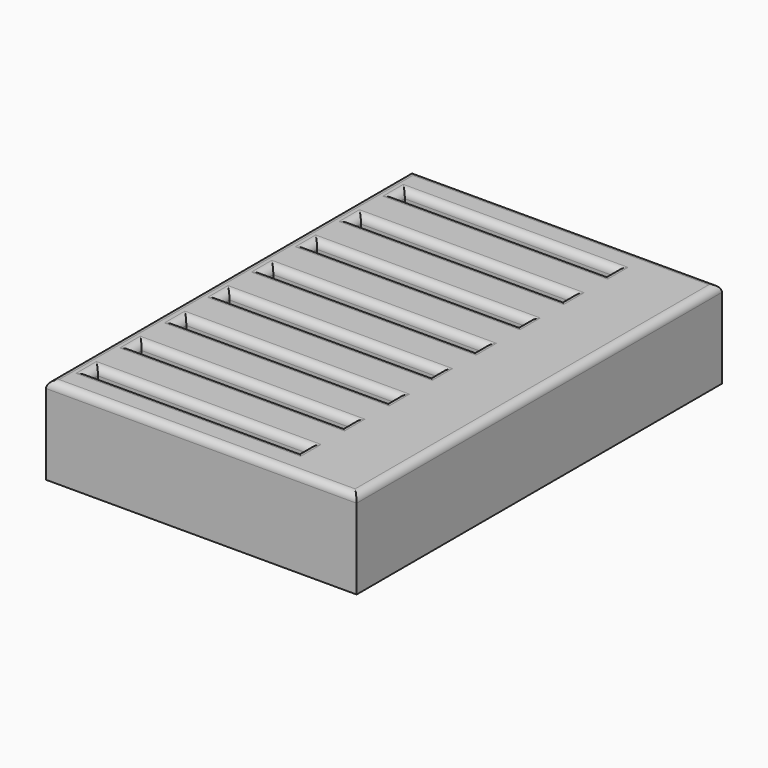
from build123d import *

# Parameters (mm, degrees)
F0_W     = 85
F0_H     = 125
F1_DEPTH = 24
F2_W     = 57.5
F2_H     = 3
F3_DEPTH = 23
F4_R     = 2


# Not quite as in the source:
# - a feature names something its author has since deleted; it is built from what else it names


with BuildPart() as f1:
    # F0 (on Top) → F1 (new body)
    with BuildSketch(Plane.XY):
        with Locations((-7.3496025801, 34.134781265)):
            Rectangle(F0_W, F0_H)
    extrude(amount=F1_DEPTH)

    # F2 (on face) → F3 (cut)
    with BuildSketch(Plane.XY.offset(24)):
        with Locations((-16.0996025801, -18.365218735)):
            Rectangle(F2_W, F2_H)
        with Locations((-16.11783728, -3.365218735)):
            Rectangle(F2_W, F2_H)
        with Locations((-15.9132478945, 11.634781265)):
            Rectangle(F2_W, F2_H)
        with Locations((-16.0996025801, 26.634781265)):
            Rectangle(F2_W, F2_H)
        with Locations((-16.0996025801, 41.634781265)):
            Rectangle(F2_W, F2_H)
        with Locations((-16.0996025801, 56.634781265)):
            Rectangle(F2_W, F2_H)
        with Locations((-16.0996025801, 71.634781265)):
            Rectangle(F2_W, F2_H)
        with Locations((-16.0996025801, 86.634781265)):
            Rectangle(F2_W, F2_H)
    extrude(amount=-F3_DEPTH, mode=Mode.SUBTRACT)

    # F4
    f4_edges = [f1.edges().sort_by_distance(p)[0] for p in [
        (-16.099603, -19.865219, 24),
        (-16.099603, -16.865219, 24),
        (12.650397, -18.365219, 24),
        (-44.849603, -18.365219, 24),
        (-16.117837, -1.865219, 24),
        (-16.117837, -4.865219, 24),
        (-44.867837, -3.365219, 24),
        (12.632163, -3.365219, 24),
        (-49.849603, 34.134781, 24),
        (-7.349603, 96.634781, 24),
        (-7.349603, -28.365219, 24),
        (35.150397, 34.134781, 24),
        (12.650397, 26.634781, 24),
        (-16.099603, 28.134781, 24),
        (-44.849603, 26.634781, 24),
        (-16.099603, 25.134781, 24),
        (12.836752, 11.634781, 24),
        (-15.913248, 13.134781, 24),
        (-44.663248, 11.634781, 24),
        (-15.913248, 10.134781, 24),
        (-16.099603, 43.134781, 24),
        (-44.849603, 41.634781, 24),
        (-16.099603, 40.134781, 24),
        (12.650397, 41.634781, 24),
        (-16.099603, 58.134781, 24),
        (-44.849603, 56.634781, 24),
        (-16.099603, 55.134781, 24),
        (12.650397, 56.634781, 24),
        (-16.099603, 73.134781, 24),
        (-44.849603, 71.634781, 24),
        (-16.099603, 70.134781, 24),
        (12.650397, 71.634781, 24),
        (-16.099603, 88.134781, 24),
        (-44.849603, 86.634781, 24),
        (-16.099603, 85.134781, 24),
        (12.650397, 86.634781, 24),
    ]]
    fillet(f4_edges, radius=F4_R)


solid = f1.part
